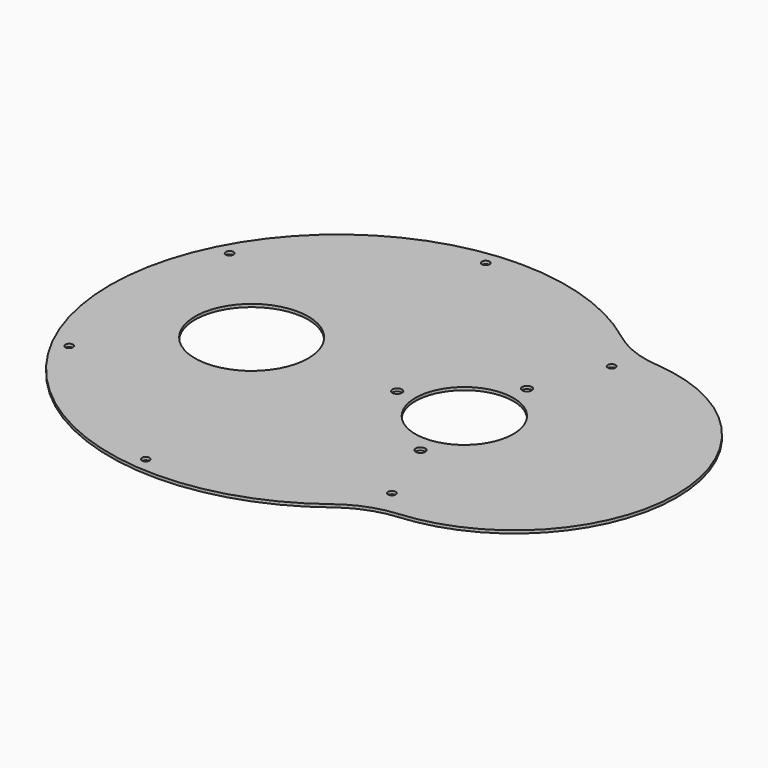
from build123d import *

# Parameters (mm, degrees)
F0_R            = 59
F0_R_2          = 51
F1_DEPTH        = 3
F2_R            = 100
F3_D            = 8
F3_COPIES_COUNT = 6
F3_COPIES_ANGLE = 280
F4_D            = 10


# Not quite as in the source:
# - a pattern or mirror of a feature is missing from the dataset's text; its kind, count and spacing are read off the source's solid


with BuildPart() as f1:
    # F0 (on Top) → F1 (new body)
    with BuildSketch(Plane.XY):
        with BuildLine():
            ThreePointArc((167.9378605318, -167.9378605318), (297.3413197874, -124.7660894685), (352.5, 0))
            ThreePointArc((352.5, 0), (297.3413197874, 124.7660894685), (167.9378605318, 167.9378605318))
            ThreePointArc((167.9378605318, 167.9378605318), (-237.5, 0), (167.9378605318, -167.9378605318))
        make_face()
        with Locations((-90, 0)):
            Circle(F0_R, mode=Mode.SUBTRACT)
        with Locations((131.5, 0)):
            Circle(F0_R_2, mode=Mode.SUBTRACT)
    extrude(amount=F1_DEPTH)

    # F2
    f2_edges = [f1.edges().sort_by_distance(p)[0] for p in [
        (167.937861, -167.937861, 1.5),
        (167.937861, 167.937861, 1.5),
    ]]
    fillet(f2_edges, radius=F2_R)

    # F3 (through all)
    with Locations(Plane(origin=(0, 0, 0), x_dir=(1, 0, 0), z_dir=(0, 0, -1))):
        with Locations((170.444888594, -143.0202431553)):
            f3 = Hole(F3_D / 2)

    # F3_copies: F3 ×6 about axis
    f3_copies_axis = Axis((0, 0, 0), (0, 0, 1))
    for i in range(1, F3_COPIES_COUNT):
        add(f3.rotate(f3_copies_axis, i * F3_COPIES_ANGLE / (F3_COPIES_COUNT - 1)), mode=Mode.SUBTRACT)

    # F4 (through all)
    with Locations(Plane(origin=(0, 0, 0), x_dir=(1, 0, 0), z_dir=(0, 0, -1))):
        with Locations((141.2421170672, -69.3187648119), (61.5, 0), (141.2421170672, 69.3187648119)):
            Hole(F4_D / 2)


solid = f1.part
